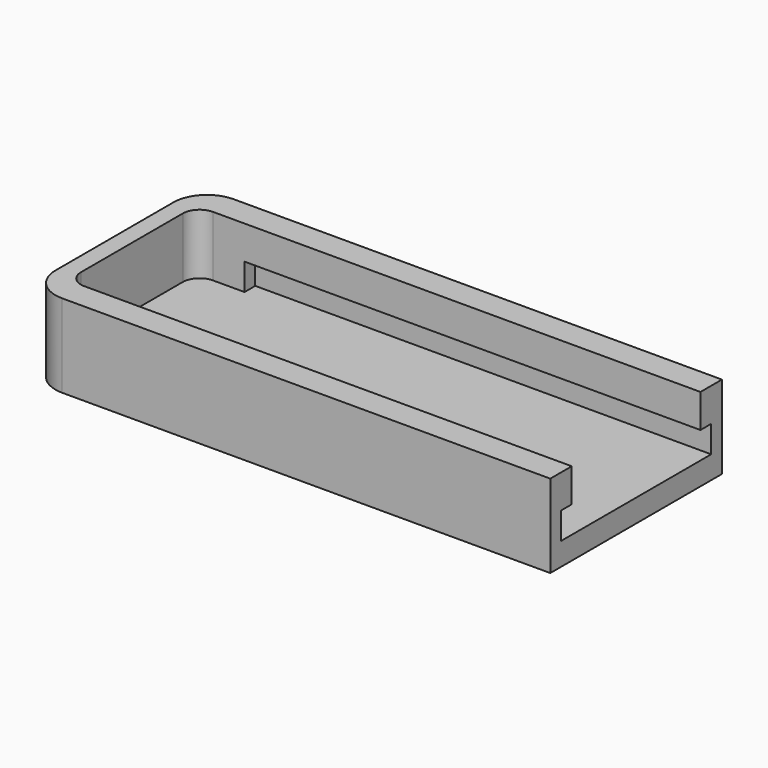
from build123d import *

# Parameters (mm, degrees)
F1_DEPTH = 7.874
F0_R     = 2.286
F2_DEPTH = 2.159
F3_W     = 17.78
F3_H     = 2.54
F4_DEPTH = 43.18


with BuildPart() as f1:
    # F0 (on Top) → F1 (new body)
    with BuildSketch(Plane.XY):
        with BuildLine():
            ThreePointArc((-24.7015, -6.985), (-23.7715640303, -9.2300640303), (-21.5265, -10.16))
            Line((-21.5265, -10.16), (24.7015, -10.16))
            Line((24.7015, -10.16), (24.7015, -7.62))
            Line((24.7015, -7.62), (-21.463, -7.62))
            ThreePointArc((-21.463, -7.62), (-22.5855320151, -7.1550320151), (-23.0505, -6.0325))
            Line((-23.0505, -6.0325), (-23.0505, 6.0325))
            ThreePointArc((-23.0505, 6.0325), (-22.5855320151, 7.1550320151), (-21.463, 7.62))
            Line((-21.463, 7.62), (24.7015, 7.62))
            Line((24.7015, 7.62), (24.7015, 10.16))
            Line((24.7015, 10.16), (-21.5265, 10.16))
            ThreePointArc((-21.5265, 10.16), (-23.7715640303, 9.2300640303), (-24.7015, 6.985))
            Line((-24.7015, 6.985), (-24.7015, -6.985))
        make_face()
    extrude(amount=F1_DEPTH)

    # F0 (on Top) → F2 (join)
    with BuildSketch(Plane.XY):
        with BuildLine():
            Line((-21.463, -7.62), (24.7015, -7.62))
            Line((24.7015, -7.62), (24.7015, 7.62))
            Line((24.7015, 7.62), (-21.463, 7.62))
            ThreePointArc((-21.463, 7.62), (-22.5855320151, 7.1550320151), (-23.0505, 6.0325))
            Line((-23.0505, 6.0325), (-23.0505, -6.0325))
            ThreePointArc((-23.0505, -6.0325), (-22.5855320151, -7.1550320151), (-21.463, -7.62))
        make_face()
        with Locations((2.9845, 0)):
            Circle(F0_R, mode=Mode.SUBTRACT)
        with Locations((2.9845, 0)):
            Circle(F0_R)
    extrude(amount=F2_DEPTH)

    # F3 (on face) → F4 (cut)
    with BuildSketch(Plane.YZ.offset(24.7015)):
        with Locations((0, 3.429)):
            Rectangle(F3_W, F3_H)
    extrude(amount=-F4_DEPTH, mode=Mode.SUBTRACT)


solid = f1.part
